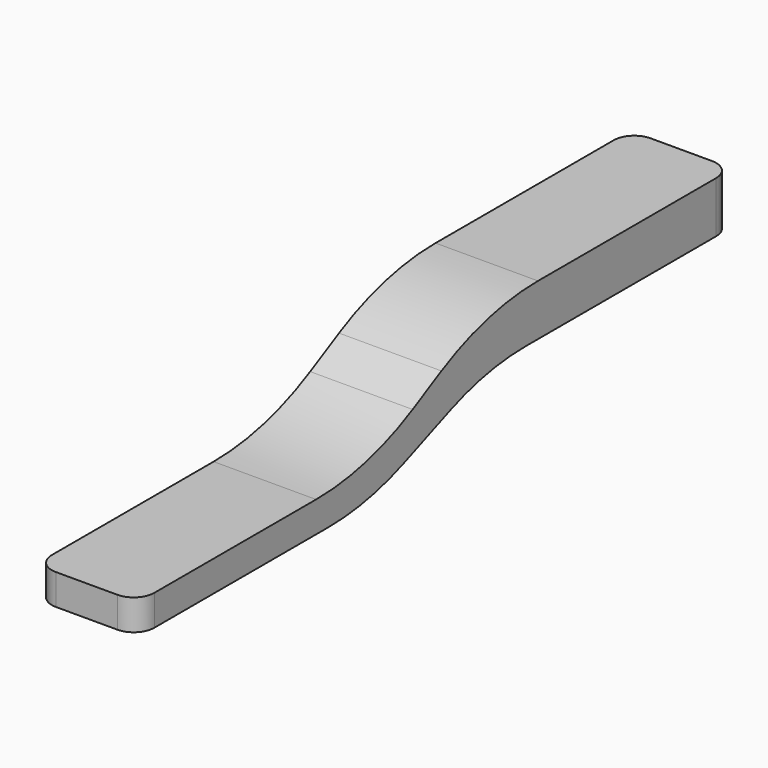
from build123d import *

# Parameters (mm, degrees)
F0_W     = 30
F0_H     = 5
F1_DEPTH = 5
F2_R     = 25
F3_R     = 2


# Not quite as in the source:
# - a feature names something its author has since deleted; it is built from what else it names


with BuildPart() as f1:
    # F0 (on Right) → F1 (new body, symmetric)
    with BuildSketch(Plane.YZ):
        Polygon((-8, 0), (0, 0), (20, 0), (20, 3), (0, 3), (-8, 3), align=None)
        Polygon((20, 3), (20, 0), (34.5558710396, 5.7734296471), (34.5558710396, 10.7734296471), align=None)
        with Locations((49.5558710396, 8.2734296471)):
            Rectangle(F0_W, F0_H)
    extrude(amount=F1_DEPTH, both=True)

    # F2
    f2_edges = [f1.edges().sort_by_distance(p)[0] for p in [
        (0, 20, 3),
        (0, 34.555871, 10.77343),
        (0, 34.555871, 5.77343),
        (0, 20, 0),
    ]]
    fillet(f2_edges, radius=F2_R)

    # F3
    f3_edges = [f1.edges().sort_by_distance(p)[0] for p in [
        (5, 64.555871, 8.27343),
        (-5, 64.555871, 8.27343),
        (5, -8, 1.5),
        (-5, -8, 1.5),
    ]]
    fillet(f3_edges, radius=F3_R)


solid = f1.part
